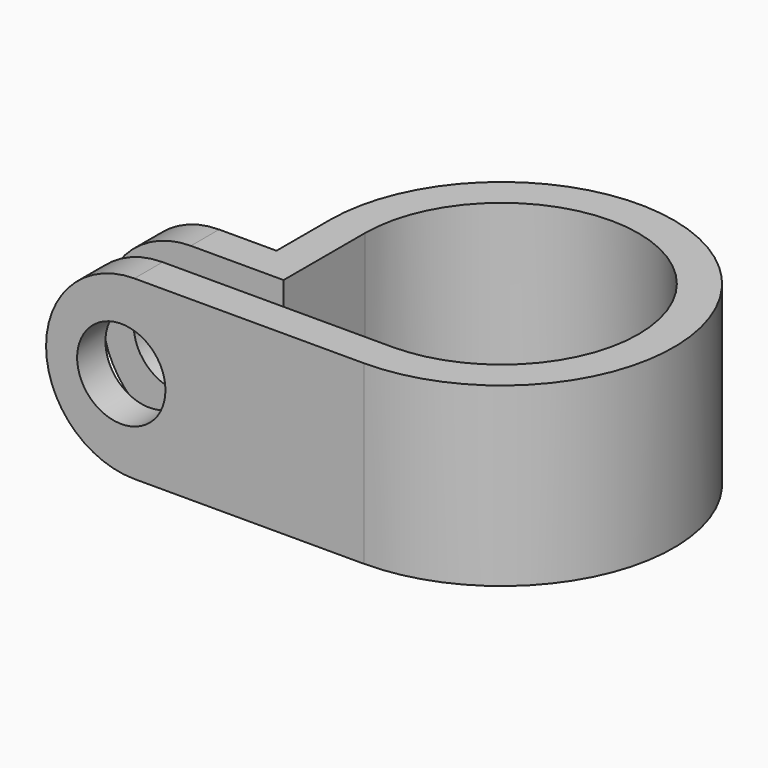
from build123d import *

# Parameters (mm, degrees)
F1_DEPTH = 10
F2_R     = 4.99999
F4_D     = 5


# Not quite as in the source:
# - a fillet or chamfer is up to 0.001 mm smaller than in the source, because OpenCascade refuses the exact size


with BuildPart() as f1:
    # F0 (on Top) → F1 (new body)
    with BuildSketch(Plane.XY):
        with BuildLine():
            ThreePointArc((-7.75, 0), (5.4800775542, 5.4800775542), (0, -7.75))
            Line((0, -7.75), (-18, -7.75))
            Line((-18, -7.75), (-18, -9.75))
            Line((-18, -9.75), (0, -9.75))
            ThreePointArc((0, -9.75), (6.8942911166, 6.8942911166), (-9.75, 0))
            Line((-9.75, 0), (-9.75, -3.75))
            Line((-9.75, -3.75), (-18, -3.75))
            Line((-18, -3.75), (-18, -5.75))
            Line((-18, -5.75), (-7.75, -5.75))
            Line((-7.75, -5.75), (-7.75, 0))
        make_face()
    extrude(amount=F1_DEPTH)

    # F2 (radius 5 in the source; OpenCascade refuses exactly that, so slightly less here)
    f2_edges = [f1.edges().sort_by_distance(p)[0] for p in [
        (-18, -4.75, 0),
        (-18, -8.75, 0),
        (-18, -8.75, 10),
        (-18, -4.75, 10),
    ]]
    fillet(f2_edges, radius=F2_R)

    # F4 (through all)
    with Locations(Plane(origin=(0, -3.75, 0), x_dir=(-1, 0, 0), z_dir=(0, 1, 0))):
        with Locations((13.740055263, 5)):
            Hole(F4_D / 2)


solid = f1.part
